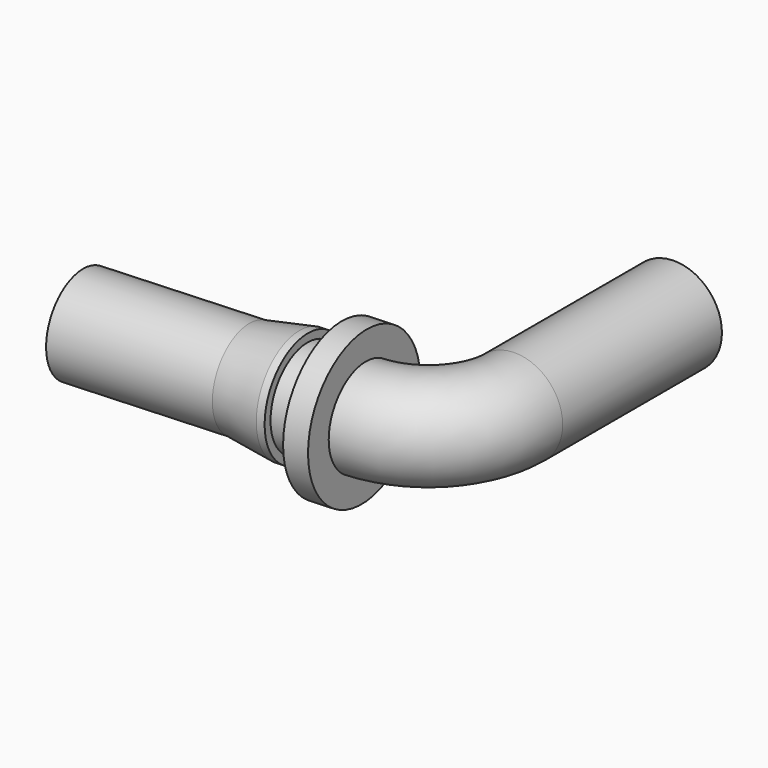
from build123d import *

# Parameters (mm, degrees)
F1_R        = 6
F1_R_2      = 4.5
F2_DEPTH    = 25
F2_FACE_R   = 6
F2_FACE_R_2 = 4.5
F4_R        = 9.5
F4_R_2      = 6
F4_R_3      = 4.5
F5_DEPTH    = 3
F6_R        = 6
F6_R_2      = 4.5
F7_DEPTH    = 4
F8_R        = 7
F8_R_2      = 6
F8_R_3      = 4.5
F9_DEPTH    = 7
F10_SIZE2   = 6
F10_SIZE    = 1
F11_R       = 6
F11_R_2     = 4.5
F12_DEPTH   = 20


with BuildPart() as f2:
    # F1 (on Front) → F2 (new body)
    with BuildSketch(Plane.XZ):
        with Locations((10.5797667056, 0)):
            Circle(F1_R)
        with Locations((10.5797667056, 0)):
            Circle(F1_R_2, mode=Mode.SUBTRACT)
    extrude(amount=-F2_DEPTH)

    # F3: sweep along a path in F0
    with BuildLine(Plane.XY) as f3_path:
        ThreePointArc((0, -4.9919255074), (3.3505289628, -3.4336417355), (4.7159582272, 0))
    # F2_face (on face) → F3 (sweep)
    with BuildSketch(Plane(origin=(10.5797667056, 0, 0), x_dir=(1, 0, 0), z_dir=(0, -1, 0))):
        Circle(F2_FACE_R)
        Circle(F2_FACE_R_2, mode=Mode.SUBTRACT)
    sweep(path=f3_path.line)

    # F4 (on face) → F5 (join)
    with BuildSketch(Plane(origin=(-0.2831251163, -0.0161098878, 0), x_dir=(0.0568083546, -0.9983851015, 0), z_dir=(-0.9983851015, -0.0568083546, 0))):
        with Locations((10.8476725327, 0)):
            Circle(F4_R)
        with Locations((10.8476725327, 0)):
            Circle(F4_R_2, mode=Mode.SUBTRACT)
        with Locations((10.8476725327, 0)):
            Circle(F4_R_2)
        with Locations((10.8476725327, 0)):
            Circle(F4_R_3, mode=Mode.SUBTRACT)
    extrude(amount=F5_DEPTH)

    # F6 (on face) → F7 (join)
    with BuildSketch(Plane(origin=(-3.2782804207, -0.1865349515, 0), x_dir=(0.0568083546, -0.9983851015, 0), z_dir=(-0.9983851015, -0.0568083546, 0))):
        with Locations((10.8476725327, 0)):
            Circle(F6_R)
        with Locations((10.8476725327, 0)):
            Circle(F6_R_2, mode=Mode.SUBTRACT)
    extrude(amount=F7_DEPTH)

    # F8 (on face) → F9 (join)
    with BuildSketch(Plane(origin=(-7.2718208266, -0.4137683698, 0), x_dir=(0.0568083546, -0.9983851015, 0), z_dir=(-0.9983851015, -0.0568083546, 0))):
        with Locations((10.8476725327, 0)):
            Circle(F8_R)
        with Locations((10.8476725327, 0)):
            Circle(F8_R_2, mode=Mode.SUBTRACT)
        with Locations((10.8476725327, 0)):
            Circle(F8_R_2)
        with Locations((10.8476725327, 0)):
            Circle(F8_R_3, mode=Mode.SUBTRACT)
    extrude(amount=F9_DEPTH)

    # F10
    f10_edges = [f2.edges().sort_by_distance(p)[0] for p in [
        (-14.041937, -4.652886, 0),
    ]]
    f10_side = f2.faces().sort_by_distance((-13.911163, -6.951178, 0))[0]
    chamfer(f10_edges, length=F10_SIZE, length2=F10_SIZE2, reference=f10_side)

    # F11 (on face) → F12 (join)
    with BuildSketch(Plane(origin=(-14.260516537, -0.8114268517, 0), x_dir=(0.0568083546, -0.9983851015, 0), z_dir=(-0.9983851015, -0.0568083546, 0))):
        with Locations((10.8476725327, 0)):
            Circle(F11_R)
        with Locations((10.8476725327, 0)):
            Circle(F11_R_2, mode=Mode.SUBTRACT)
    extrude(amount=F12_DEPTH)


solid = f2.part
